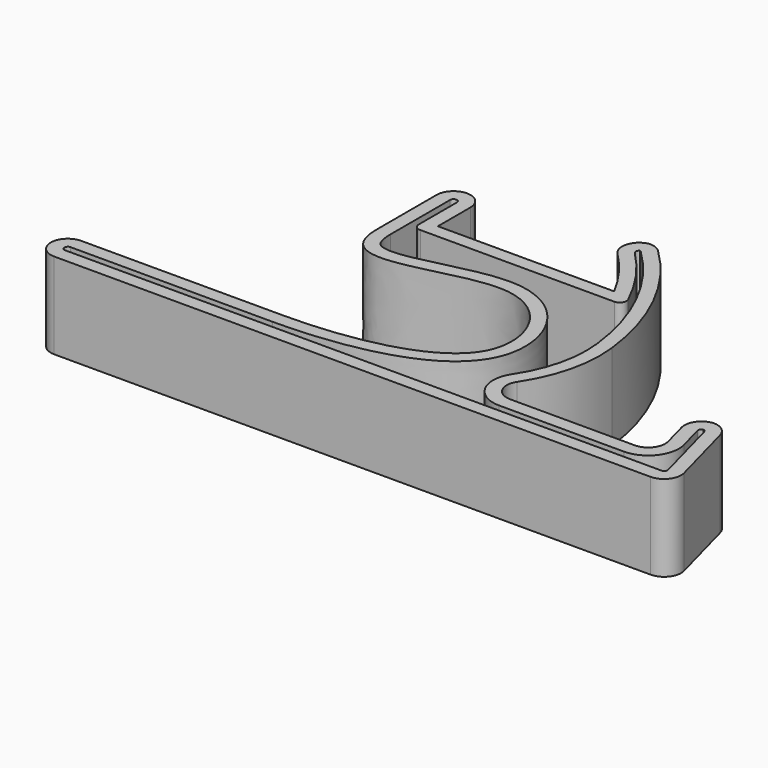
from build123d import *

# Parameters (mm, degrees)
F1_DEPTH     = 12.7
F2_R         = 20
F3_R         = 2.5
F5_DEPTH     = 12.7
F6_F1_R      = 2.5
F6_T2_DEPTH  = 40.6809764225
F6_T4_DEPTH  = 18.842488162
F6_T6_DEPTH  = 26.9902706656
F6_T8_DEPTH  = 23.634012634
F6_T10_DEPTH = 28.9903171605
F6_T12_DEPTH = 22.2915873497
F8_DEPTH     = 12.7010001
F9_R         = 1


# Not quite as in the source:
# - a fillet or chamfer that OpenCascade refuses, or shapes differently, is made with other operations: its cross-section is extruded or revolved along the edge and cut away or added
# - the dataset's text gives a spline's control points without its knots; the knots are read off the source's solid
# - a feature names something its author has since deleted; it is built from what else it names


with BuildPart() as f1:
    # F0 (on Top) → F1 (new body)
    with BuildSketch(Plane.XY):
        with BuildLine():
            Line((26, 0), (0, 0))
            Line((0, 0), (0, 8.865468193))
            Line((0, 8.865468193), (-5, 8.1942165867))
            Line((-5, 8.1942165867), (-5, -5))
            add(Edge.make_bspline(
                [(-5, -5), (-5, -15.501089584), (19.0256931719, 0.3567569325), (30.1756624289, -24.9177696597), (9.6326051711, -28.4992713986), (0, -28.4992713986)],
                knots=[0, 0, 0, 0, 0.3417333641, 0.6271848675, 1, 1, 1, 1], degree=3))
            Line((0, -28.4992713986), (-32.2831194267, -28.4992713986))
            Line((-32.2831194267, -28.4992713986), (-32.2831194267, -33.5))
            Line((-32.2831194267, -33.5), (30.1841822348, -33.5))
            ThreePointArc((30.1841822348, -33.5), (34.3653616818, -9.4887703025), (22.7052848786, 11.9136599824))
            Line((22.7052848786, 11.9136599824), (16.333817732, 11.058288471))
            ThreePointArc((16.333817732, 11.058288471), (21.8099348194, 6.0912209154), (26, 0))
        make_face()
    extrude(amount=F1_DEPTH)

    # F2
    f2_edges = [f1.edges().sort_by_distance(p)[0] for p in [
        (30.184182, -33.5, 6.35),
    ]]
    fillet(f2_edges, radius=F2_R)

    # F3
    f3_edges = [f1.edges().sort_by_distance(p)[0] for p in [
        (-32.283119, -28.499271, 6.35),
        (-32.283119, -33.5, 6.35),
    ]]
    fillet(f3_edges, radius=F3_R)

    # F4 (on face) → F5 (join, through all)
    with BuildSketch(Plane.XY.offset(12.7)):
        with BuildLine():
            ThreePointArc((27.96768626, -28.5), (21.8099975165, -32.2082869339), (14.7389297046, -33.5))
            Line((14.7389297046, -33.5), (61.4277839948, -33.5))
            Line((61.4277839948, -33.5), (57.4085461083, -18.5))
            Line((57.4085461083, -18.5), (52.4085461083, -18.5))
            Line((52.4085461083, -18.5), (55.0880380326, -28.5))
            Line((55.0880380326, -28.5), (27.96768626, -28.5))
        make_face()
    extrude(amount=-F5_DEPTH)

    # F6: fillet of radius 2.5 on 9 edges, made by hand

    # F6_f1
    f6_f1_edges = [f1.edges().sort_by_distance(p)[0] for p in [
        (55.0880380326, -28.5, 6.35),
        (27.96768626, -28.5, 6.35),
    ]]
    fillet(f6_f1_edges, radius=F6_F1_R)

    # F6_s3 → F6_t2 (cut)
    with BuildSketch(Plane.XY.offset(-13.9904882113)):
        with BuildLine():
            ThreePointArc((21.8802540946, 11.8028993346), (19.8462095939, 10.1306076425), (20.4378221029, 7.5646982182))
            Line((20.4378221029, 7.5646982182), (20.4023206317, 7.5294896178))
            ThreePointArc((20.4023206317, 7.5294896178), (18.4270917304, 9.3599763345), (16.3047287677, 11.0176211358))
            Line((16.3047287677, 11.0176211358), (16.3271649007, 11.1078438929))
            Line((16.3271649007, 11.1078438929), (21.8736012633, 11.8524547564))
            Line((21.8736012633, 11.8524547564), (21.8802540946, 11.8028993346))
        make_face()
    extrude(amount=F6_T2_DEPTH, mode=Mode.SUBTRACT)

    # F6_s5 → F6_t4 (cut)
    with BuildSketch(Plane.XY.offset(-3.071244081)):
        with BuildLine():
            ThreePointArc((23.6017049623, 11.0736376813), (22.6439697377, 11.6526732309), (21.5295641298, 11.7558190941))
            Line((21.5295641298, 11.7558190941), (21.5229112985, 11.805374516))
            Line((21.5229112985, 11.805374516), (22.6986320473, 11.9632154042))
            Line((22.6986320473, 11.9632154042), (22.7388634855, 11.9507069413))
            ThreePointArc((22.7388634855, 11.9507069413), (23.1911705381, 11.5338539314), (23.6364949476, 11.1095494749))
            Line((23.6364949476, 11.1095494749), (23.6017049623, 11.0736376813))
        make_face()
    extrude(amount=F6_T4_DEPTH, mode=Mode.SUBTRACT)

    # F6_s7 → F6_t6 (cut)
    with BuildSketch(Plane.XY.offset(-7.1451353328)):
        with BuildLine():
            ThreePointArc((0, 6.0074140599), (-0.8540358317, 7.8891159376), (-2.8326415652, 8.4851851529))
            Line((-2.8326415652, 8.4851851529), (-2.8392943966, 8.5347405747))
            Line((-2.8392943966, 8.5347405747), (0.05, 8.9226292757))
            Line((0.05, 8.9226292757), (0.05, 6.0074140599))
            Line((0.05, 6.0074140599), (0, 6.0074140599))
        make_face()
    extrude(amount=F6_T6_DEPTH, mode=Mode.SUBTRACT)

    # F6_s9 → F6_t8 (cut)
    with BuildSketch(Plane.XY.offset(-5.467006317)):
        with BuildLine():
            ThreePointArc((-5, 6.0074140599), (-4.3817018777, 7.6533782282), (-2.8326415652, 8.4851851529))
            Line((-2.8326415652, 8.4851851529), (-2.8392943966, 8.5347405747))
            Line((-2.8392943966, 8.5347405747), (-5.05, 8.2379526372))
            Line((-5.05, 8.2379526372), (-5.05, 6.0074140599))
            Line((-5.05, 6.0074140599), (-5, 6.0074140599))
        make_face()
    extrude(amount=F6_T8_DEPTH, mode=Mode.SUBTRACT)

    # F6_s11 → F6_t10 (cut)
    with BuildSketch(Plane.XY.offset(-8.1451585803)):
        with BuildLine():
            ThreePointArc((53.2517949747, -21.6470476128), (53.6832261897, -19.4780964275), (55.6666095404, -18.5))
            Line((55.6666095404, -18.5), (55.6666095404, -18.45))
            Line((55.6666095404, -18.45), (52.3433848397, -18.45))
            Line((52.3433848397, -18.45), (53.2034986834, -21.659988565))
            Line((53.2034986834, -21.659988565), (53.2517949747, -21.6470476128))
        make_face()
        with BuildLine():
            ThreePointArc((60.5845351284, -30.3529523872), (60.1531039134, -32.5219035725), (58.1697205627, -33.5))
            Line((58.1697205627, -33.5), (58.1697205627, -33.55))
            Line((58.1697205627, -33.55), (61.4929452634, -33.55))
            Line((61.4929452634, -33.55), (60.6328314197, -30.340011435))
            Line((60.6328314197, -30.340011435), (60.5845351284, -30.3529523872))
        make_face()
    extrude(amount=F6_T10_DEPTH, mode=Mode.SUBTRACT)

    # F6_s13 → F6_t12 (cut)
    with BuildSketch(Plane.XY.offset(-4.7957936749)):
        with BuildLine():
            ThreePointArc((55.4902286384, -18.5), (57.0121322109, -19.0166166493), (57.9050432041, -20.3529523872))
            Line((57.9050432041, -20.3529523872), (57.9533394954, -20.340011435))
            Line((57.9533394954, -20.340011435), (57.4469124577, -18.45))
            Line((57.4469124577, -18.45), (55.4902286384, -18.45))
            Line((55.4902286384, -18.45), (55.4902286384, -18.5))
        make_face()
    extrude(amount=F6_T12_DEPTH, mode=Mode.SUBTRACT)

    # F7 (on face) → F8 (cut, through all)
    with BuildSketch(Plane.XY.offset(12.7)):
        with BuildLine():
            ThreePointArc((29.7055592517, -23.5), (32.2419928899, -17.7003308359), (32.6137914787, -11.3811992641))
            ThreePointArc((32.6137914787, -11.3811992641), (29.2247911313, 0.0253055143), (22.2101055485, 9.6371659372))
            ThreePointArc((22.2101055485, 9.6371659372), (22.1014246136, 9.7171087134), (21.9753262516, 9.7650836669))
            ThreePointArc((21.9753262516, 9.7650836669), (21.7183035133, 9.3984672393), (21.8578809484, 8.9730422369))
            ThreePointArc((21.8578809484, 8.9730422369), (26.0386131908, 3.842878095), (29.1463264613, -2))
            Line((29.1463264613, -2), (-2, -2))
            Line((-2, -2), (-2, 6.0074140599))
            ThreePointArc((-2, 6.0074140599), (-2.5, 6.5074140599), (-3, 6.0074140599))
            Line((-3, 6.0074140599), (-3, -5))
            add(Edge.make_bspline(
                [(-3, -5), (-3, -5.404140573), (-2.9535206775, -6.111730584), (-2.7830041154, -6.875987521), (-2.564643096, -7.3683542221), (-2.3428373272, -7.6618764819), (-2.0989458439, -7.8647572616), (-1.7531611295, -8.0401633725), (-1.2459815159, -8.1790601552), (-0.3440798429, -8.2781860542), (1.157546462, -8.1953279523), (3.3631658748, -7.7906434324), (5.8269244847, -7.1947906743), (8.4429674732, -6.5355344882), (10.6811834802, -6.0444678372), (12.4770095179, -5.7571106504), (13.8215291533, -5.6139097987), (14.9373630322, -5.5730515161), (15.8246825888, -5.6002925023), (16.711140415, -5.6733419698), (17.7831779174, -5.8546184706), (19.4042120726, -6.3223383811), (21.2370067018, -7.2150209517), (23.0804927803, -8.6794041339), (24.5488406424, -10.4367523194), (25.6361291023, -12.4002034469), (26.3373039298, -14.4964250815), (26.6400413993, -16.6605918961), (26.539829502, -18.4691962922), (26.2289975159, -19.8823696529), (25.874215812, -20.916067708), (25.394599863, -21.9019329523), (24.6140705268, -23.1184814805), (23.4044179516, -24.4619258009), (21.6679279509, -25.8096686692), (19.0480735214, -27.3074025498), (15.3019375322, -28.7039408164), (10.3139811914, -29.7893961788), (5.1001645384, -30.3820957029), (1.6619121378, -30.4992713986), (0, -30.4992713986)],
                knots=[0, 0, 0, 0, 0.015625, 0.03125, 0.046875, 0.0625, 0.078125, 0.09375, 0.109375, 0.125, 0.15625, 0.1875, 0.21875, 0.25, 0.28125, 0.296875, 0.3125, 0.328125, 0.3359375, 0.34375, 0.359375, 0.375, 0.40625, 0.4375, 0.46875, 0.5, 0.53125, 0.5625, 0.59375, 0.609375, 0.625, 0.640625, 0.65625, 0.6875, 0.71875, 0.75, 0.8125, 0.875, 0.9375, 1, 1, 1, 1], degree=3))
            Line((0, -30.4992713986), (-29.7831194267, -30.4992713986))
            ThreePointArc((-29.7831194267, -30.4992713986), (-30.1366728173, -30.645718008), (-30.2831194267, -30.9992713986))
            Line((-30.2831194267, -30.9992713986), (-30.2831194267, -31))
            ThreePointArc((-30.2831194267, -31), (-30.1366728173, -31.3535533906), (-29.7831194267, -31.5))
            Line((-29.7831194267, -31.5), (58.1697205627, -31.5))
            ThreePointArc((58.1697205627, -31.5), (58.5663972328, -31.3043807145), (58.6526834758, -30.8705904774))
            Line((58.6526834758, -30.8705904774), (55.9731915515, -20.8705904774))
            ThreePointArc((55.9731915515, -20.8705904774), (55.8285350068, -20.6318304724), (55.5784190894, -20.5078390057))
            ThreePointArc((55.5784190894, -20.5078390057), (55.2445413964, -20.731935676), (55.1836466273, -21.1294095226))
            Line((55.1836466273, -21.1294095226), (56.1766408188, -24.835314297))
            ThreePointArc((56.1766408188, -24.835314297), (55.4000646318, -28.7394264305), (51.8299746005, -30.5))
            Line((51.8299746005, -30.5), (33.4472166385, -30.5))
            ThreePointArc((33.4472166385, -30.5), (29.4785896719, -28.1213203436), (29.7055592517, -23.5))
        make_face()
    extrude(amount=-F8_DEPTH, mode=Mode.SUBTRACT)

    # F9
    f9_edges = [f1.edges().sort_by_distance(p)[0] for p in [
        (29.146326, -2, 6.35),
        (-2, -2, 6.35),
    ]]
    fillet(f9_edges, radius=F9_R)


solid = f1.part
